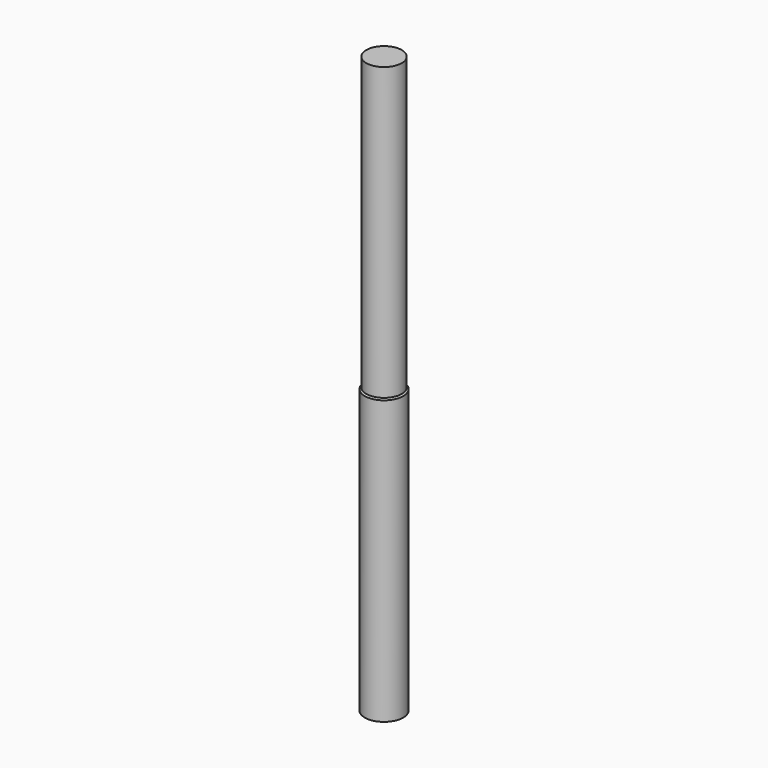
from build123d import *

# Parameters (mm, degrees)
F0_R        = 5.08
F1_DEPTH    = 76.2
F2_R        = 4.699
F3_DEPTH    = 76.2
F4_S5_R     = 4.699
F4_T6_DEPTH = 9


# Not quite as in the source:
# - a fillet or chamfer that OpenCascade refuses, or shapes differently, is made with other operations: its cross-section is extruded or revolved along the edge and cut away or added


with BuildPart() as f1:
    # F0 (on Top) → F1 (new body)
    with BuildSketch(Plane.XY):
        Circle(F0_R)
    extrude(amount=-F1_DEPTH)

    # F2 (on face) → F3 (join)
    with BuildSketch(Plane.XY):
        Circle(F2_R)
    extrude(amount=F3_DEPTH)

    # F4: chamfer of 1.27 on 1 edges, made by hand


with BuildPart() as f4_tool2:
    # F4_s3 → F4_t4 (revolve)
    with BuildSketch(Plane.XZ):
        Polygon((5.08, -1.27), (3.81, 0), (5.08, 0), align=None)
    revolve(axis=Axis((0, 0, 0), (0, 0, 1)))

    # F4_s5 → F4_t6 (cut, symmetric)
    with BuildSketch(Plane.XY.offset(-0.6)):
        Circle(F4_S5_R)
    extrude(amount=F4_T6_DEPTH, both=True, mode=Mode.SUBTRACT)


with BuildPart() as f1_1:
    add(f1.part)

    # F4_t1: cut F4_tool2
    add(f4_tool2.part, mode=Mode.SUBTRACT)


solid = f1_1.part
